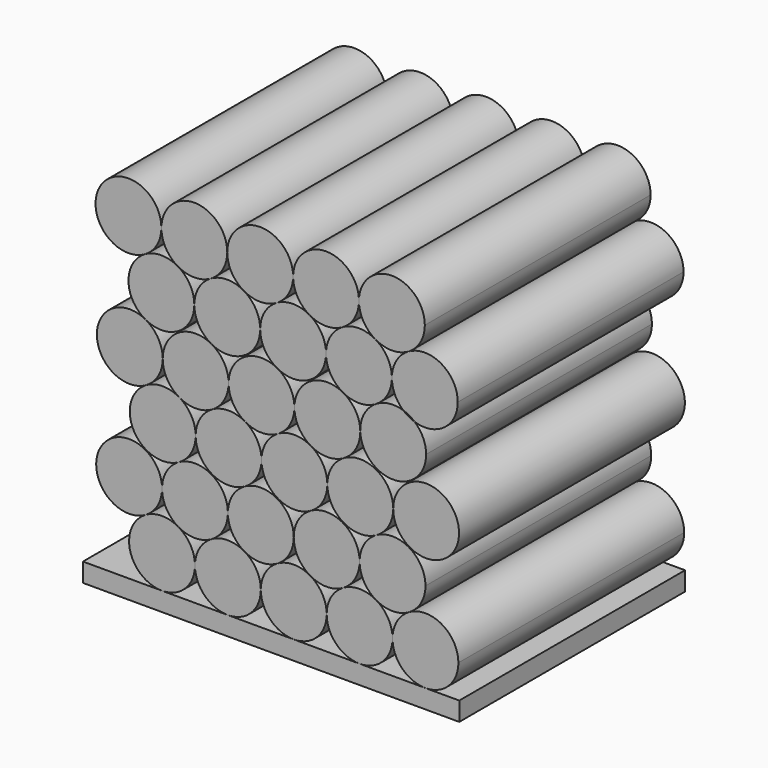
from build123d import *

# Parameters (mm, degrees)
F1_DEPTH = 76.2


# Not quite as in the source:
# - a feature names something its author has since deleted; it is built from what else it names


with BuildPart() as f1:
    # F0 (on Front) → F1 (new body)
    with BuildSketch(Plane.XZ):
        with BuildLine():
            ThreePointArc((-29.4477027383, -25.4555717693), (-23.1615234536, -22.851751054), (-20.5577027383, -16.5655717693))
            ThreePointArc((-20.5577027383, -16.5655717693), (-21.7487368667, -12.1205718246), (-25.0027026277, -8.8666059935))
            ThreePointArc((-25.0027026277, -8.8666059935), (-29.4477026803, -7.6755717693), (-33.8927027485, -8.8666059355))
            ThreePointArc((-33.8927027485, -8.8666059355), (-38.0347833325, -18.8664730859), (-29.4477027383, -25.4555717693))
        make_face()
    extrude(amount=F1_DEPTH)


with BuildPart() as f1b:
    # F0 (on Front) → F1, piece 2 (new body)
    with BuildSketch(Plane.XZ):
        with BuildLine():
            ThreePointArc((-16.1127027426, -8.8666059321), (-19.3666685792, -12.1205717714), (-20.5577027383, -16.5655717693))
            ThreePointArc((-20.5577027383, -16.5655717693), (-17.9538820218, -22.8517510553), (-11.6677027346, -25.4555717693))
            ThreePointArc((-11.6677027346, -25.4555717693), (-5.3815234523, -22.8517510527), (-2.7777027383, -16.5655717693))
            ThreePointArc((-2.7777027383, -16.5655717693), (-3.9687368512, -12.1205718515), (-7.2227025739, -8.8666060246))
            ThreePointArc((-7.2227025739, -8.8666060246), (-11.6677026458, -7.6755717693), (-16.1127027426, -8.8666059321))
        make_face()
    extrude(amount=F1_DEPTH)


with BuildPart() as f1c:
    # F0 (on Front) → F1, piece 3 (new body)
    with BuildSketch(Plane.XZ):
        with BuildLine():
            ThreePointArc((-29.4477027383, -1.16764009), (-28.256668546, -5.6126401453), (-25.0027026277, -8.8666059935))
            ThreePointArc((-25.0027026277, -8.8666059935), (-20.5577026769, -10.05764009), (-16.1127027426, -8.8666059321))
            ThreePointArc((-16.1127027426, -8.8666059321), (-12.8587368999, -5.6126400921), (-11.6677027383, -1.16764009))
            ThreePointArc((-11.6677027383, -1.16764009), (-16.0669411864, 6.5047233453), (-24.9107085164, 6.5837108049))
            ThreePointArc((-24.9107085164, 6.5837108049), (-28.2300661736, 3.323121462), (-29.4477027383, -1.16764009))
        make_face()
    extrude(amount=F1_DEPTH)


with BuildPart() as f1d:
    # F0 (on Front) → F1, piece 4 (new body)
    with BuildSketch(Plane.XZ):
        with BuildLine():
            ThreePointArc((50.7462852537, 14.3350614461), (41.8562852537, 23.2250614461), (32.9662852537, 14.3350614461))
            ThreePointArc((32.9662852537, 14.3350614461), (41.8562852537, 5.4450614461), (50.7462852537, 14.3350614461))
        make_face()
    extrude(amount=F1_DEPTH)


with BuildPart() as f1e:
    # F0 (on Front) → F1, piece 5 (new body)
    with BuildSketch(Plane.XZ):
        Polygon((-11.6677027346, -25.4555717693), (-29.4477027383, -25.4555717693), (-50.8, -25.4555717693), (-50.8, -30.5355717693), (50.8, -30.5355717693), (50.8, -25.4555717693), (41.6722971921, -25.4555717693), (23.8922972402, -25.4555717693), (6.1122972617, -25.4555717693), align=None)
    extrude(amount=F1_DEPTH)


with BuildPart() as f1f:
    # F0 (on Front) → F1, piece 6 (new body)
    with BuildSketch(Plane.XZ):
        with BuildLine():
            ThreePointArc((-29.4477027383, -1.16764009), (-46.036668575, 3.2773599151), (-33.8927027485, -8.8666059355))
            ThreePointArc((-33.8927027485, -8.8666059355), (-30.6387369016, -5.6126400951), (-29.4477027383, -1.16764009))
        make_face()
    extrude(amount=F1_DEPTH)


with BuildPart() as f1g:
    # F0 (on Front) → F1, piece 7 (new body)
    with BuildSketch(Plane.XZ):
        with BuildLine():
            ThreePointArc((-11.6677027383, -1.16764009), (-10.4766685305, -5.6126401722), (-7.2227025739, -8.8666060246))
            ThreePointArc((-7.2227025739, -8.8666060246), (-2.7777025673, -10.05764009), (1.6672973934, -8.8666058536))
            ThreePointArc((1.6672973934, -8.8666058536), (4.9212631394, -5.6126400241), (6.1122972617, -1.16764009))
            ThreePointArc((6.1122972617, -1.16764009), (1.7130586982, 6.5047234129), (-7.1307087496, 6.583710674))
            ThreePointArc((-7.1307087496, 6.583710674), (-10.4500662412, 3.3231213466), (-11.6677027383, -1.16764009))
        make_face()
    extrude(amount=F1_DEPTH)


with BuildPart() as f1h:
    # F0 (on Front) → F1, piece 8 (new body)
    with BuildSketch(Plane.XZ):
        with BuildLine():
            ThreePointArc((1.6672973934, -8.8666058536), (-1.5866685399, -12.1205717034), (-2.7777027383, -16.5655717693))
            ThreePointArc((-2.7777027383, -16.5655717693), (-0.1738820231, -22.851751054), (6.1122972617, -25.4555717693))
            ThreePointArc((6.1122972617, -25.4555717693), (12.3984765464, -22.851751054), (15.0022972617, -16.5655717693))
            ThreePointArc((15.0022972617, -16.5655717693), (13.8112631619, -12.1205718742), (10.5572974715, -8.8666060508))
            ThreePointArc((10.5572974715, -8.8666060508), (6.1122974589, -7.6755717693), (1.6672973934, -8.8666058536))
        make_face()
    extrude(amount=F1_DEPTH)


with BuildPart() as f1i:
    # F0 (on Front) → F1, piece 9 (new body)
    with BuildSketch(Plane.XZ):
        with BuildLine():
            ThreePointArc((-33.7087146145, 22.0340273618), (-36.9890099597, 9.935980421), (-24.9107085164, 6.5837108049))
            ThreePointArc((-24.9107085164, 6.5837108049), (-21.5913511801, 9.8443001178), (-20.3737147463, 14.3350614461))
            ThreePointArc((-20.3737147463, 14.3350614461), (-21.564748866, 18.7800613757), (-24.8187146054, 22.0340272044))
            ThreePointArc((-24.8187146054, 22.0340272044), (-29.2637145889, 23.2250614461), (-33.7087146145, 22.0340273618))
        make_face()
    extrude(amount=F1_DEPTH)


with BuildPart() as f1j:
    # F0 (on Front) → F1, piece 10 (new body)
    with BuildSketch(Plane.XZ):
        with BuildLine():
            ThreePointArc((-20.3737147463, 14.3350614461), (-15.97447619, 6.6626979475), (-7.1307087496, 6.583710674))
            ThreePointArc((-7.1307087496, 6.583710674), (-3.8113512476, 9.8443000024), (-2.5937147463, 14.3350614461))
            ThreePointArc((-2.5937147463, 14.3350614461), (-3.7847488029, 18.7800612665), (-7.0387143871, 22.0340270784))
            ThreePointArc((-7.0387143871, 22.0340270784), (-11.483714467, 23.2250614461), (-15.9287146218, 22.0340273576))
            ThreePointArc((-15.9287146218, 22.0340273576), (-19.18268055, 18.7800615083), (-20.3737147463, 14.3350614461))
        make_face()
    extrude(amount=F1_DEPTH)


with BuildPart() as f1k:
    # F0 (on Front) → F1, piece 11 (new body)
    with BuildSketch(Plane.XZ):
        with BuildLine():
            ThreePointArc((19.4472973755, -8.8666058639), (16.1933314549, -12.1205717124), (15.0022972617, -16.5655717693))
            ThreePointArc((15.0022972617, -16.5655717693), (17.6061179693, -22.8517510464), (23.8922972402, -25.4555717693))
            ThreePointArc((23.8922972402, -25.4555717693), (30.1784765388, -22.8517510616), (32.7822972617, -16.5655717693))
            ThreePointArc((32.7822972617, -16.5655717693), (31.5912630633, -12.1205717034), (28.3372971299, -8.8666058536))
            ThreePointArc((28.3372971299, -8.8666058536), (23.8922972513, -7.6755717693), (19.4472973755, -8.8666058639))
        make_face()
    extrude(amount=F1_DEPTH)


with BuildPart() as f1l:
    # F0 (on Front) → F1, piece 12 (new body)
    with BuildSketch(Plane.XZ):
        with BuildLine():
            ThreePointArc((-33.8871814008, 37.5322747084), (-47.0431253896, 29.6306289991), (-33.7087146145, 22.0340273618))
            ThreePointArc((-33.7087146145, 22.0340273618), (-30.4547488686, 25.2879931913), (-29.2637147463, 29.7329931254))
            ThreePointArc((-29.2637147463, 29.7329931254), (-30.5064413289, 34.2663483155), (-33.8871814008, 37.5322747084))
        make_face()
    extrude(amount=F1_DEPTH)


with BuildPart() as f1m:
    # F0 (on Front) → F1, piece 13 (new body)
    with BuildSketch(Plane.XZ):
        with BuildLine():
            ThreePointArc((6.1122972617, -1.16764009), (7.3033314826, -5.6126401949), (10.5572974715, -8.8666060508))
            ThreePointArc((10.5572974715, -8.8666060508), (15.0022974485, -10.05764009), (19.4472973755, -8.8666058639))
            ThreePointArc((19.4472973755, -8.8666058639), (22.7012631342, -5.6126400331), (23.8922972617, -1.16764009))
            ThreePointArc((23.8922972617, -1.16764009), (19.4930587398, 6.5047233886), (10.6492913344, 6.5837107211))
            ThreePointArc((10.6492913344, 6.5837107211), (7.3299337831, 3.3231213881), (6.1122972617, -1.16764009))
        make_face()
    extrude(amount=F1_DEPTH)


with BuildPart() as f1n:
    # F0 (on Front) → F1, piece 14 (new body)
    with BuildSketch(Plane.XZ):
        with BuildLine():
            ThreePointArc((1.8512849925, 22.0340271349), (-1.4026806613, 18.7800613155), (-2.5937147463, 14.3350614461))
            ThreePointArc((-2.5937147463, 14.3350614461), (1.8055238515, 6.6626979231), (10.6492913344, 6.5837107211))
            ThreePointArc((10.6492913344, 6.5837107211), (13.9686487767, 9.8443000439), (15.1862852537, 14.3350614461))
            ThreePointArc((15.1862852537, 14.3350614461), (13.9952512129, 18.7800612391), (10.7412856677, 22.0340270467))
            ThreePointArc((10.7412856677, 22.0340270467), (6.2962853419, 23.2250614461), (1.8512849925, 22.0340271349))
        make_face()
    extrude(amount=F1_DEPTH)


with BuildPart() as f1o:
    # F0 (on Front) → F1, piece 15 (new body)
    with BuildSketch(Plane.XZ):
        with BuildLine():
            ThreePointArc((37.2272973436, -8.8666058823), (33.9733314457, -12.1205717283), (32.7822972617, -16.5655717693))
            ThreePointArc((32.7822972617, -16.5655717693), (35.3861179524, -22.8517510294), (41.6722971921, -25.4555717693))
            ThreePointArc((41.6722971921, -25.4555717693), (47.9584765218, -22.8517510786), (50.5622972617, -16.5655717693))
            ThreePointArc((50.5622972617, -16.5655717693), (46.1172973026, -8.8666059533), (37.2272973436, -8.8666058823))
        make_face()
    extrude(amount=F1_DEPTH)


with BuildPart() as f1p:
    # F0 (on Front) → F1, piece 16 (new body)
    with BuildSketch(Plane.XZ):
        with BuildLine():
            ThreePointArc((-29.2637147463, 29.7329931254), (-28.0726805453, 25.2879930549), (-24.8187146054, 22.0340272044))
            ThreePointArc((-24.8187146054, 22.0340272044), (-20.3737145931, 20.8429931254), (-15.9287146218, 22.0340273576))
            ThreePointArc((-15.9287146218, 22.0340273576), (-12.6747488707, 25.2879931876), (-11.4837147463, 29.7329931254))
            ThreePointArc((-11.4837147463, 29.7329931254), (-12.7264413663, 34.2663483787), (-16.1071815297, 37.532274779))
            ThreePointArc((-16.1071815297, 37.532274779), (-24.9070699995, 37.3802665053), (-29.2637147463, 29.7329931254))
        make_face()
    extrude(amount=F1_DEPTH)


with BuildPart() as f1q:
    # F0 (on Front) → F1, piece 17 (new body)
    with BuildSketch(Plane.XZ):
        with BuildLine():
            ThreePointArc((-34.0656474485, 53.0305219473), (-38.5100582284, 45.2291923281), (-33.8871814008, 37.5322747084))
            ThreePointArc((-33.8871814008, 37.5322747084), (-25.087292623, 37.6842824761), (-20.7306475802, 45.3315560316))
            ThreePointArc((-20.7306475802, 45.3315560316), (-21.9216817786, 49.7765560975), (-25.1756477119, 53.0305219473))
            ThreePointArc((-25.1756477119, 53.0305219473), (-29.6206475802, 54.2215560316), (-34.0656474485, 53.0305219473))
        make_face()
    extrude(amount=F1_DEPTH)


with BuildPart() as f1r:
    # F0 (on Front) → F1, piece 18 (new body)
    with BuildSketch(Plane.XZ):
        with BuildLine():
            ThreePointArc((-11.4837147463, 29.7329931254), (-10.2926804822, 25.2879929458), (-7.0387143871, 22.0340270784))
            ThreePointArc((-7.0387143871, 22.0340270784), (-2.5937146897, 20.8429931254), (1.8512849925, 22.0340271349))
            ThreePointArc((1.8512849925, 22.0340271349), (5.1052510179, 25.2879929948), (6.2962852537, 29.7329931254))
            ThreePointArc((6.2962852537, 29.7329931254), (5.053558772, 34.2663481453), (1.6728189462, 37.5322745186))
            ThreePointArc((1.6728189462, 37.5322745186), (-7.1270697662, 37.3802666437), (-11.4837147463, 29.7329931254))
        make_face()
    extrude(amount=F1_DEPTH)


with BuildPart() as f1s:
    # F0 (on Front) → F1, piece 19 (new body)
    with BuildSketch(Plane.XZ):
        with BuildLine():
            ThreePointArc((23.8922972617, -1.16764009), (25.083331384, -5.6126400241), (28.3372971299, -8.8666058536))
            ThreePointArc((28.3372971299, -8.8666058536), (32.7822972329, -10.05764009), (37.2272973436, -8.8666058823))
            ThreePointArc((37.2272973436, -8.8666058823), (40.481263125, -5.612640049), (41.6722972617, -1.16764009))
            ThreePointArc((41.6722972617, -1.16764009), (37.2730586761, 6.5047234258), (28.4292912057, 6.5837106489))
            ThreePointArc((28.4292912057, 6.5837106489), (25.1099337459, 3.3231213244), (23.8922972617, -1.16764009))
        make_face()
    extrude(amount=F1_DEPTH)


with BuildPart() as f1t:
    # F0 (on Front) → F1, piece 20 (new body)
    with BuildSketch(Plane.XZ):
        with BuildLine():
            ThreePointArc((-29.6206475802, 60.7294877109), (-46.2096134579, 65.174487645), (-34.0656474485, 53.0305219473))
            ThreePointArc((-34.0656474485, 53.0305219473), (-30.8116817025, 56.2844877768), (-29.6206475802, 60.7294877109))
        make_face()
    extrude(amount=F1_DEPTH)


with BuildPart() as f1u:
    # F0 (on Front) → F1, piece 21 (new body)
    with BuildSketch(Plane.XZ):
        with BuildLine():
            ThreePointArc((-16.2856475789, 53.030521872), (-19.5396134195, 49.7765560323), (-20.7306475802, 45.3315560316))
            ThreePointArc((-20.7306475802, 45.3315560316), (-19.4879211732, 40.7982011377), (-16.1071815297, 37.532274779))
            ThreePointArc((-16.1071815297, 37.532274779), (-7.3072926862, 37.6842824386), (-2.9506475802, 45.3315560316))
            ThreePointArc((-2.9506475802, 45.3315560316), (-4.1416817444, 49.7765560383), (-7.3956475937, 53.030521879))
            ThreePointArc((-7.3956475937, 53.030521879), (-11.8406475872, 54.2215560316), (-16.2856475789, 53.030521872))
        make_face()
    extrude(amount=F1_DEPTH)


with BuildPart() as f1v:
    # F0 (on Front) → F1, piece 22 (new body)
    with BuildSketch(Plane.XZ):
        with BuildLine():
            ThreePointArc((19.6312850473, 22.0340271665), (16.3773193545, 18.7800613429), (15.1862852537, 14.3350614461))
            ThreePointArc((15.1862852537, 14.3350614461), (19.5855237879, 6.6626979604), (28.4292912057, 6.5837106489))
            ThreePointArc((28.4292912057, 6.5837106489), (31.7486487394, 9.8442999802), (32.9662852537, 14.3350614461))
            ThreePointArc((32.9662852537, 14.3350614461), (28.5212851505, 22.0340273453), (19.6312850473, 22.0340271665))
        make_face()
    extrude(amount=F1_DEPTH)


with BuildPart() as f1w:
    # F0 (on Front) → F1, piece 23 (new body)
    with BuildSketch(Plane.XZ):
        with BuildLine():
            ThreePointArc((6.2962852537, 29.7329931254), (7.4873195336, 25.2879929184), (10.7412856677, 22.0340270467))
            ThreePointArc((10.7412856677, 22.0340270467), (15.1862853735, 20.8429931254), (19.6312850473, 22.0340271665))
            ThreePointArc((19.6312850473, 22.0340271665), (22.8852510338, 25.2879930222), (24.0762852537, 29.7329931254))
            ThreePointArc((24.0762852537, 29.7329931254), (24.0756958986, 29.8353571176), (24.0739279113, 29.9377075375))
            ThreePointArc((24.0739279113, 29.9377075375), (22.7808523572, 34.3541023548), (19.4528186617, 37.5322746743))
            ThreePointArc((19.4528186617, 37.5322746743), (10.6529300943, 37.380266561), (6.2962852537, 29.7329931254))
        make_face()
    extrude(amount=F1_DEPTH)


with BuildPart() as f1x:
    # F0 (on Front) → F1, piece 24 (new body)
    with BuildSketch(Plane.XZ):
        with BuildLine():
            ThreePointArc((-29.6206475802, 60.7294877109), (-28.4296134579, 56.2844877768), (-25.1756477119, 53.0305219473))
            ThreePointArc((-25.1756477119, 53.0305219473), (-20.7306476555, 51.8394877109), (-16.2856475789, 53.030521872))
            ThreePointArc((-16.2856475789, 53.030521872), (-13.0316817402, 56.2844877115), (-11.8406475802, 60.7294877109))
            ThreePointArc((-11.8406475802, 60.7294877109), (-20.7306475802, 69.6194877109), (-29.6206475802, 60.7294877109))
        make_face()
    extrude(amount=F1_DEPTH)


with BuildPart() as f1y:
    # F0 (on Front) → F1, piece 25 (new body)
    with BuildSketch(Plane.XZ):
        with BuildLine():
            ThreePointArc((1.4943525052, 53.0305219205), (-1.7596133952, 49.7765560743), (-2.9506475802, 45.3315560316))
            ThreePointArc((-2.9506475802, 45.3315560316), (-1.7079210348, 40.7982009043), (1.6728189462, 37.5322745186))
            ThreePointArc((1.6728189462, 37.5322745186), (10.4727075471, 37.684282577), (14.8293524198, 45.3315560316))
            ThreePointArc((14.8293524198, 45.3315560316), (13.6383183056, 49.7765559516), (10.3843525797, 53.0305217789))
            ThreePointArc((10.3843525797, 53.0305217789), (5.9393525614, 54.2215560316), (1.4943525052, 53.0305219205))
        make_face()
    extrude(amount=F1_DEPTH)


with BuildPart() as f1z:
    # F0 (on Front) → F1, piece 26 (new body)
    with BuildSketch(Plane.XZ):
        with BuildLine():
            ThreePointArc((14.8293524198, 45.3315560316), (16.0720788825, 40.7982010438), (19.4528186617, 37.5322746743))
            ThreePointArc((19.4528186617, 37.5322746743), (23.9240666623, 36.4439133701), (28.3404616426, 37.7369889241))
            ThreePointArc((28.3404616426, 37.7369889241), (31.4689898626, 40.9755005333), (32.6093524198, 45.3315560316))
            ThreePointArc((32.6093524198, 45.3315560316), (31.4183182214, 49.7765560975), (28.1643522881, 53.0305219473))
            ThreePointArc((28.1643522881, 53.0305219473), (23.7193523445, 54.2215560316), (19.2743524211, 53.030521872))
            ThreePointArc((19.2743524211, 53.030521872), (16.0203865805, 49.7765560323), (14.8293524198, 45.3315560316))
        make_face()
    extrude(amount=F1_DEPTH)


with BuildPart() as f1ba:
    # F0 (on Front) → F1, piece 27 (new body)
    with BuildSketch(Plane.XZ):
        with BuildLine():
            ThreePointArc((5.9393524198, 60.7294877109), (-2.9506475802, 69.6194877109), (-11.8406475802, 60.7294877109))
            ThreePointArc((-11.8406475802, 60.7294877109), (-10.6496134237, 56.2844877176), (-7.3956475937, 53.030521879))
            ThreePointArc((-7.3956475937, 53.030521879), (-2.9506475387, 51.8394877109), (1.4943525052, 53.0305219205))
            ThreePointArc((1.4943525052, 53.0305219205), (4.7483182841, 56.2844877536), (5.9393524198, 60.7294877109))
        make_face()
    extrude(amount=F1_DEPTH)


with BuildPart() as f1bb:
    # F0 (on Front) → F1, piece 28 (new body)
    with BuildSketch(Plane.XZ):
        with BuildLine():
            ThreePointArc((28.3404616426, 37.7369889241), (25.1622892007, 34.4089553656), (24.0739279113, 29.9377075375))
            ThreePointArc((24.0739279113, 29.9377075375), (33.0639344137, 21.2530109938), (41.8515705761, 30.1424216405))
            ThreePointArc((41.8515705761, 30.1424216405), (41.0453728657, 33.8416432535), (38.7730012752, 36.8699303346))
            ThreePointArc((38.7730012752, 36.8699303346), (37.1432968477, 37.5819186303), (35.6879217207, 38.6040473375))
            ThreePointArc((35.6879217207, 38.6040473375), (31.9197095764, 38.9711602626), (28.3404616426, 37.7369889241))
        make_face()
    extrude(amount=F1_DEPTH)


with BuildPart() as f1bc:
    # F0 (on Front) → F1, piece 29 (new body)
    with BuildSketch(Plane.XZ):
        with BuildLine():
            ThreePointArc((23.7193524198, 60.7294877109), (14.8293524198, 69.6194877109), (5.9393524198, 60.7294877109))
            ThreePointArc((5.9393524198, 60.7294877109), (7.1303866263, 56.2844876309), (10.3843525797, 53.0305217789))
            ThreePointArc((10.3843525797, 53.0305217789), (14.8293525129, 51.8394877109), (19.2743524211, 53.030521872))
            ThreePointArc((19.2743524211, 53.030521872), (22.5283182598, 56.2844877115), (23.7193524198, 60.7294877109))
        make_face()
    extrude(amount=F1_DEPTH)


with BuildPart() as f1bd:
    # F0 (on Front) → F1, piece 30 (new body)
    with BuildSketch(Plane.XZ):
        with BuildLine():
            ThreePointArc((32.6093524198, 45.3315560316), (33.4155501302, 41.6323344185), (35.6879217207, 38.6040473375))
            ThreePointArc((35.6879217207, 38.6040473375), (37.3176261482, 37.8920590418), (38.7730012752, 36.8699303346))
            ThreePointArc((38.7730012752, 36.8699303346), (46.7336068235, 38.1458284527), (50.3893524198, 45.3315560316))
            ThreePointArc((50.3893524198, 45.3315560316), (45.9443524857, 53.0305218332), (37.0543525515, 53.0305219473))
            ThreePointArc((37.0543525515, 53.0305219473), (33.8003866182, 49.7765560975), (32.6093524198, 45.3315560316))
        make_face()
    extrude(amount=F1_DEPTH)


with BuildPart() as f1be:
    # F0 (on Front) → F1, piece 31 (new body)
    with BuildSketch(Plane.XZ):
        with BuildLine():
            ThreePointArc((41.4993524198, 60.7294877109), (32.6093524198, 69.6194877109), (23.7193524198, 60.7294877109))
            ThreePointArc((23.7193524198, 60.7294877109), (24.9103865421, 56.2844877768), (28.1643522881, 53.0305219473))
            ThreePointArc((28.1643522881, 53.0305219473), (32.6093524198, 51.8394877109), (37.0543525515, 53.0305219473))
            ThreePointArc((37.0543525515, 53.0305219473), (40.3083182975, 56.2844877768), (41.4993524198, 60.7294877109))
        make_face()
    extrude(amount=F1_DEPTH)


solid = Compound([f1.part, f1b.part, f1c.part, f1d.part, f1e.part, f1f.part, f1g.part, f1h.part, f1i.part, f1j.part, f1k.part, f1l.part, f1m.part, f1n.part, f1o.part, f1p.part, f1q.part, f1r.part, f1s.part, f1t.part, f1u.part, f1v.part, f1w.part, f1x.part, f1y.part, f1z.part, f1ba.part, f1bb.part, f1bc.part, f1bd.part, f1be.part])
